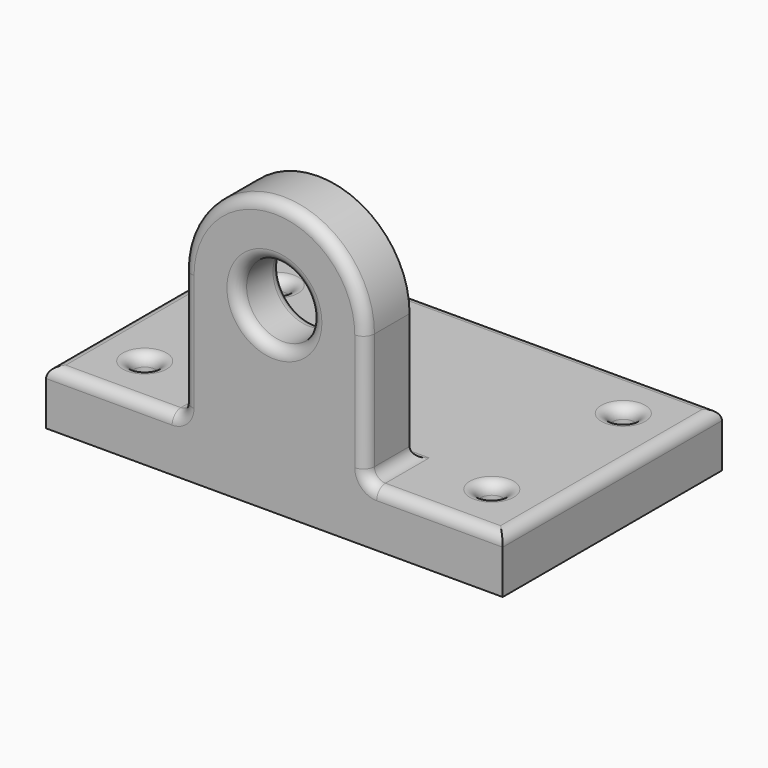
from build123d import *

# Parameters (mm, degrees)
F0_W     = 125
F0_H     = 75
F1_DEPTH = 15
F3_DEPTH = 15
F4_R     = 3
F5_DEPTH = 25
F6_R     = 3


with BuildPart() as f1:
    # F0 (on Top) → F1 (new body)
    with BuildSketch(Plane.XY):
        Rectangle(F0_W, F0_H)
    extrude(amount=F1_DEPTH)

    # F2 (on face) → F3 (join)
    with BuildSketch(Plane.XZ.offset(37.5)):
        with BuildLine():
            Line((10, 50), (25, 50))
            ThreePointArc((25, 50), (0, 75), (-25, 50))
            Line((-25, 50), (-10, 50))
            ThreePointArc((-10, 50), (0, 60), (10, 50))
        make_face()
        with BuildLine():
            ThreePointArc((-25, 50), (0, 25), (25, 50))
            Line((25, 50), (10, 50))
            ThreePointArc((10, 50), (0, 40), (-10, 50))
            Line((-10, 50), (-25, 50))
        make_face()
        with BuildLine():
            Line((25, 15), (25, 50))
            ThreePointArc((25, 50), (0, 25), (-25, 50))
            Line((-25, 50), (-25, 15))
            Line((-25, 15), (25, 15))
        make_face()
    extrude(amount=-F3_DEPTH)

    # F4 (on face) → F5 (cut)
    with BuildSketch(Plane.XY.offset(15)):
        with Locations((-47.5, 22.5)):
            Circle(F4_R)
        with Locations((-47.5, -22.5)):
            Circle(F4_R)
        with Locations((47.5, 22.5)):
            Circle(F4_R)
        with Locations((47.5, -22.5)):
            Circle(F4_R)
    extrude(amount=-F5_DEPTH, mode=Mode.SUBTRACT)

    # F6
    f6_edges = [f1.edges().sort_by_distance(p)[0] for p in [
        (-62.5, 0, 15),
        (0, 37.5, 15),
        (-43.75, -37.5, 15),
        (62.5, 0, 15),
        (-25, -30, 15),
        (43.75, -37.5, 15),
        (0, -22.5, 15),
        (25, -30, 15),
        (-50.5, -22.5, 15),
        (44.5, -22.5, 15),
        (-50.5, 22.5, 15),
        (44.5, 22.5, 15),
        (-10, -37.5, 50),
        (-10, -22.5, 50),
        (-25, -37.5, 32.5),
        (0, -37.5, 75),
        (25, -37.5, 32.5),
    ]]
    fillet(f6_edges, radius=F6_R)


solid = f1.part
